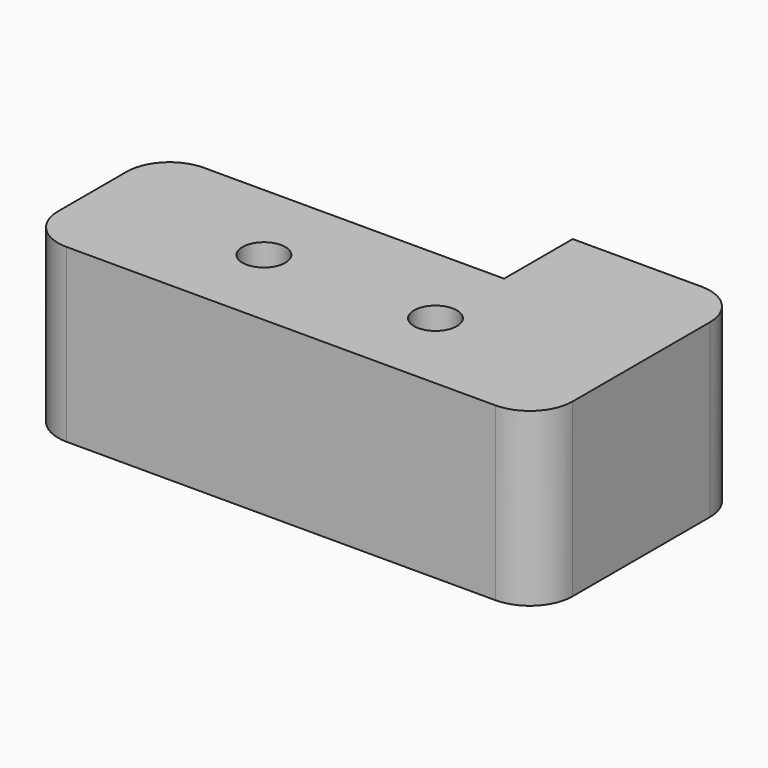
from build123d import *

# Parameters (mm, degrees)
F1_DEPTH = 50.8
F2_R     = 12.7
F4_D     = 12.7


# Not quite as in the source:
# - ends of sketch curves that miss each other by under 0.0002 mm in the source are joined


with BuildPart() as f1:
    # F0 (on Top) → F1 (new body)
    with BuildSketch(Plane.XY):
        Polygon((0, 50.8), (0, 0), (152.4000018835, 0), (152.4, 76.2), (101.6, 76.2), (101.6, 50.8), align=None)
    extrude(amount=F1_DEPTH)

    # F2
    f2_edges = [f1.edges().sort_by_distance(p)[0] for p in [
        (0, 0, 25.4),
        (0, 50.8, 25.4),
        (152.4, 76.2, 25.4),
        (152.400002, 0, 25.4),
    ]]
    fillet(f2_edges, radius=F2_R)

    # F4 (through all)
    with Locations(Plane.XY.offset(50.8)):
        with Locations((50.8, 25.4), (101.6, 25.4)):
            Hole(F4_D / 2)


solid = f1.part
